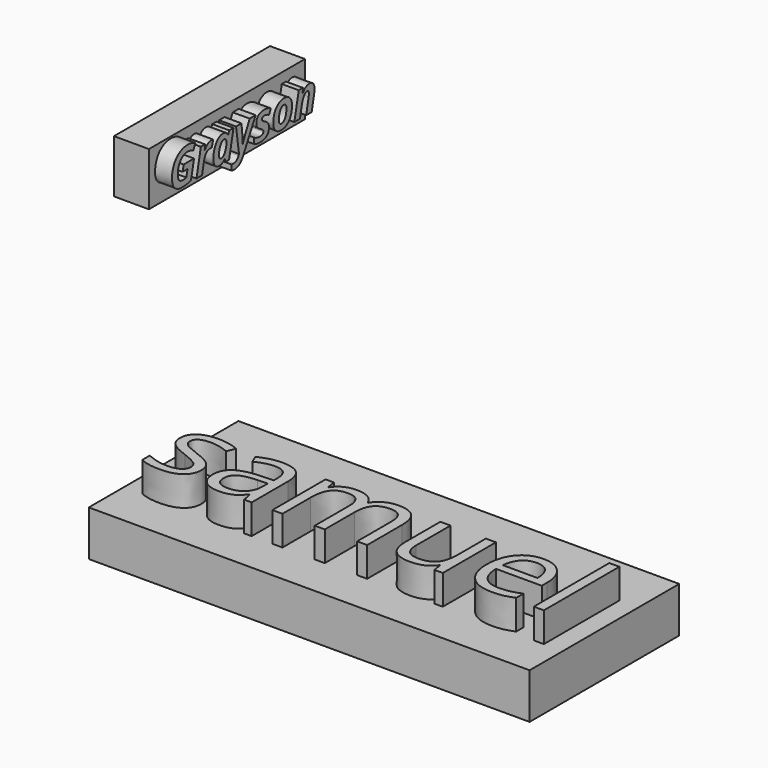
from build123d import *

# Parameters (mm, degrees)
F0_W         = 640.5609846115
F0_H         = 66.0727694631
F1_DEPTH     = 271.78
F2_TEXT_SIZE = 180.4372295737
F3_DEPTH     = 43.18
F4_W         = 187.8906935453
F4_H         = 56.2516450882
F5_DEPTH     = 50.8
F7_DEPTH     = 52.578
F8_DEPTH     = 42.926
F9_DEPTH     = 20.828
F6_TEXT_SIZE = 68.5718324449
F10_DEPTH    = 24.638


# Not quite as in the source:
# - Text() gives the source's letters only with a copy of the font that has no kerning and outlines rounded to 1/6400 em; it was checked with that copy


with BuildPart() as f1:
    # F0 (on Front) → F1 (new body)
    with BuildSketch(Plane.XZ):
        with Locations((486.4482879639, -33.0363847315)):
            Rectangle(F0_W, F0_H)
    extrude(amount=F1_DEPTH)

    # F2 (on face) → F3 (join)
    with BuildSketch(Plane.XY):
        with Locations((182.8095465899, -211.4400714636)):
            Text('samuel', F2_TEXT_SIZE, font='Open Sans', text_align=(TextAlign.LEFT, TextAlign.BOTTOM))
    extrude(amount=F3_DEPTH)


with BuildPart() as f5:
    # F4 (on Right) → F5 (new body)
    with BuildSketch(Plane.YZ):
        with Locations((128.2410547137, 289.7024452686)):
            Rectangle(F4_W, F4_H)
    extrude(amount=F5_DEPTH)

    # F7 (add): a face of the model
    f7_faces = [f5.faces().sort_by_distance(p)[0] for p in [
        (25.4, 34.2957079411, 289.7024452686),
    ]]
    extrude(f7_faces, amount=F7_DEPTH)

    # F8 (add): a face of the model
    f8_faces = [f5.faces().sort_by_distance(p)[0] for p in [
        (25.4, 222.1864014864, 289.7024452686),
    ]]
    extrude(f8_faces, amount=F8_DEPTH)

    # F9 (add): a face of the model
    f9_faces = [f5.faces().sort_by_distance(p)[0] for p in [
        (25.4, 123.4150547137, 261.5766227245),
    ]]
    extrude(f9_faces, amount=F9_DEPTH)

    # F6 (on face) → F10 (join)
    with BuildSketch(Plane.YZ.offset(50.8)):
        with Locations((-11.2511143088, 265.5215859413)):
            Text('Grayson', F6_TEXT_SIZE, font='Open Sans', font_style=FontStyle.BOLDITALIC, text_align=(TextAlign.LEFT, TextAlign.BOTTOM))
    extrude(amount=F10_DEPTH)


solid = Compound([f1.part, f5.part])
